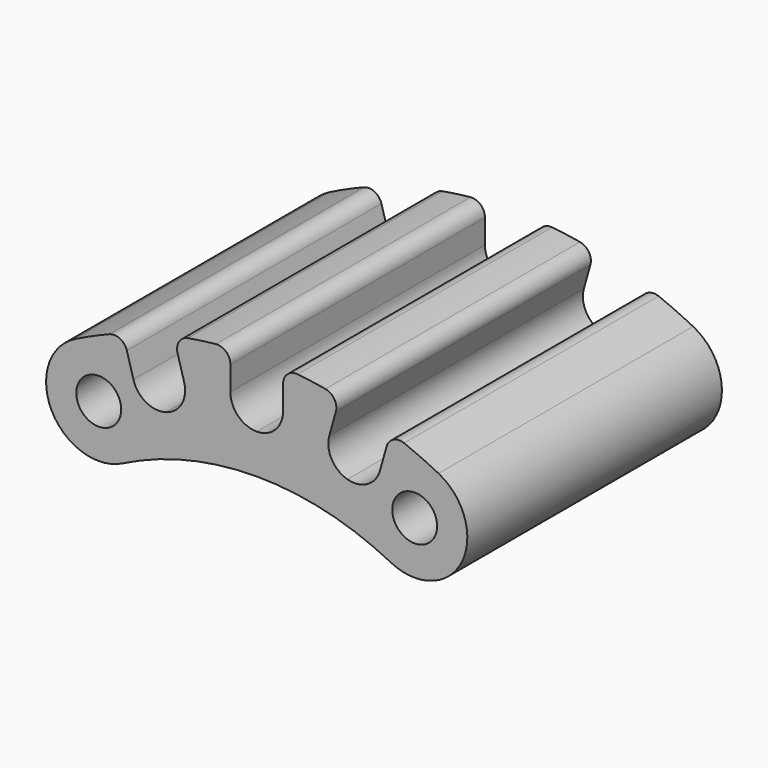
from build123d import *

# Parameters (mm, degrees)
F0_R     = 1.35255
F1_DEPTH = 19.18716
F2_W     = 3.175
F2_H     = 3.96875
F3_DEPTH = 19.18716
F4_R     = 1.58749
F5_R     = 0.79375
F6_R     = 0.79375
F7_DEPTH = 55


# Not quite as in the source:
# - a fillet or chamfer is up to 0.001 mm smaller than in the source, because OpenCascade refuses the exact size
# - an extrude ends at something that could not be found from the text; its depth is read off the source's solid


with BuildPart() as f1:
    # F0 (on Front) → F1 (new body)
    with BuildSketch(Plane.XZ):
        with BuildLine():
            ThreePointArc((-8.0873006088, 15.9239409983), (0, 17.8599084), (8.0873006088, 15.9239409983))
            ThreePointArc((8.0873006088, 15.9239409983), (12.3558382964, 17.3170799036), (10.9626993912, 21.5856175912))
            ThreePointArc((10.9626993912, 21.5856175912), (0, 24.2099084), (-10.9626993912, 21.5856175912))
            ThreePointArc((-10.9626993912, 21.5856175912), (-12.3558382964, 17.3170799036), (-8.0873006088, 15.9239409983))
        make_face()
        with Locations((-9.525, 18.7547792948)):
            Circle(F0_R, mode=Mode.SUBTRACT)
        with Locations((9.525, 18.7547792948)):
            Circle(F0_R, mode=Mode.SUBTRACT)
    extrude(amount=F1_DEPTH)

    # F2 (on face) → F3 (cut, through all)
    with BuildSketch(Plane.XZ.offset(19.18716)):
        Polygon((-8.0765705738, 22.8781299226), (-7.0031118134, 19.0573102654), (-3.9464560877, 19.9160772737), (-5.0199148481, 23.7368969308), align=None)
        Polygon((8.0765705738, 22.8781299226), (5.0199148481, 23.7368969308), (3.9464560877, 19.9160772737), (7.0031118134, 19.0573102654), align=None)
        with Locations((0, 22.2255334)):
            Rectangle(F2_W, F2_H)
    extrude(amount=-F3_DEPTH, mode=Mode.SUBTRACT)

    # F4 (radius 1.5875 in the source; OpenCascade refuses exactly that, so slightly less here)
    f4_edges = [f1.edges().sort_by_distance(p)[0] for p in [
        (-7.003112, -9.59358, 19.05731),
        (-3.946456, -9.59358, 19.916077),
        (-1.5875, -9.59358, 20.241158),
        (1.5875, -9.59358, 20.241158),
        (3.946456, -9.59358, 19.916077),
        (7.003112, -9.59358, 19.05731),
    ]]
    fillet(f4_edges, radius=F4_R)

    # F5
    f5_edges = [f1.edges().sort_by_distance(p)[0] for p in [
        (-8.062478, -9.59358, 22.827968),
        (-5.005822, -9.59358, 23.686735),
        (-1.5875, -9.59358, 24.157804),
        (1.5875, -9.59358, 24.157804),
        (5.005822, -9.59358, 23.686735),
        (8.062478, -9.59358, 22.827968),
    ]]
    fillet(f5_edges, radius=F5_R)

    # F6 (on Top) → F7 (cut, through all)
    with BuildSketch(Plane.XY):
        with Locations((0, -9.59358)):
            Circle(F6_R)
    extrude(amount=F7_DEPTH, mode=Mode.SUBTRACT)


solid = f1.part
